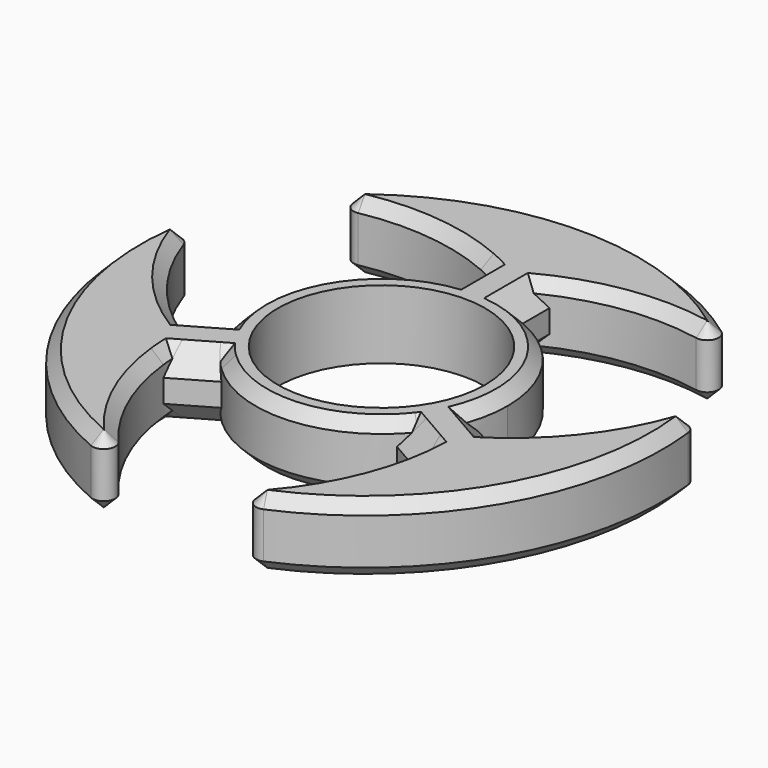
from build123d import *

# Parameters (mm, degrees)
F0_R          = 11.5
F1_DEPTH      = 7.62
F2_R          = 1.27
F3_SIZE       = 2.54
F4_T2_ANGLE   = 73.3947953897
F4_T4_ANGLE   = 73.3947953897
F4_T6_ANGLE   = 73.3947953897
F4_T8_ANGLE   = 73.3947953897
F4_T10_ANGLE  = 73.3947953897
F4_T12_ANGLE  = 73.3947953897
F4_T14_ANGLE  = 88.3467597363
F4_T16_ANGLE  = 88.3467597363
F4_T18_ANGLE  = 88.3467597363
F4_T20_ANGLE  = 88.3467597363
F4_T22_ANGLE  = 88.3467597363
F4_T24_ANGLE  = 88.3467597363
F4_T28_ANGLE  = 24.0059301026
F4_T33_ANGLE  = 24.0059301026
F4_T38_ANGLE  = 24.0059301026
F4_T43_ANGLE  = 24.0059301026
F4_T48_ANGLE  = 24.0059301026
F4_T53_ANGLE  = 24.0059301026
F4_T58_ANGLE  = 24.0059301026
F4_T63_ANGLE  = 24.0059301026
F4_T68_ANGLE  = 24.0059301026
F4_T73_ANGLE  = 24.0059301026
F4_T78_ANGLE  = 24.0059301026
F4_T83_ANGLE  = 24.0059301026
F4_T88_ANGLE  = 24.0059301026
F4_T93_ANGLE  = 24.0059301026
F4_T98_ANGLE  = 24.0059301026
F4_T103_ANGLE = 24.0059301026
F4_T108_ANGLE = 24.0059301026
F4_T113_ANGLE = 24.0059301026
F4_T118_ANGLE = 24.0059301026
F4_T123_ANGLE = 24.0059301026
F4_T128_ANGLE = 24.0059301026
F4_T133_ANGLE = 24.0059301026
F4_T138_ANGLE = 24.0059301026
F4_T143_ANGLE = 24.0059301026
F4_T146_ANGLE = 154.1156868675
F4_T148_ANGLE = 154.1156868949
F4_T150_ANGLE = 34.3912629475
F4_T154_ANGLE = 13.7891656583
F4_T157_ANGLE = 34.3912629475
F4_T161_ANGLE = 13.7891656583
F4_T164_ANGLE = 154.1156868675
F4_T166_ANGLE = 154.1156868675
F4_T168_ANGLE = 34.3912629475
F4_T172_ANGLE = 13.7891656583
F4_T175_ANGLE = 34.3912629475
F4_T179_ANGLE = 13.7891656583
F4_T182_ANGLE = 154.1156868675
F4_T184_ANGLE = 154.1156868675
F4_T186_ANGLE = 34.3912629475
F4_T190_ANGLE = 13.7891656583
F4_T193_ANGLE = 34.3912629475
F4_T197_ANGLE = 13.7891656583
F4_T200_ANGLE = 154.1156868675
F4_T202_ANGLE = 154.1156868949
F4_T204_ANGLE = 34.3912629475
F4_T208_ANGLE = 13.7891656583
F4_T211_ANGLE = 34.3912629475
F4_T215_ANGLE = 13.7891656583
F4_T218_ANGLE = 154.1156868675
F4_T220_ANGLE = 154.1156868675
F4_T222_ANGLE = 34.3912629475
F4_T226_ANGLE = 13.7891656583
F4_T229_ANGLE = 34.3912629475
F4_T233_ANGLE = 13.7891656583
F4_T236_ANGLE = 154.1156868675
F4_T238_ANGLE = 154.1156868675
F4_T240_ANGLE = 34.3912629475
F4_T244_ANGLE = 13.7891656583
F4_T247_ANGLE = 34.3912629475
F4_T251_ANGLE = 13.7891656583


# Not quite as in the source:
# - a fillet or chamfer that OpenCascade refuses, or shapes differently, is made with other operations: its cross-section is extruded or revolved along the edge and cut away or added


with BuildPart() as f1:
    # F0 (on Top) → F1 (new body)
    with BuildSketch(Plane.XY):
        with BuildLine():
            ThreePointArc((13.5447422652, -3.4206515417), (13.8632779213, -1.7234921751), (13.97, 0))
            ThreePointArc((13.97, 0), (11.144204772, 8.4242269675), (3.81, 13.4404166602))
            ThreePointArc((3.81, 13.4404166602), (0, 13.97), (-3.81, 13.4404166602))
            ThreePointArc((-3.81, 13.4404166602), (-12.0983748909, 6.985), (-13.5447422652, -3.4206515417))
            ThreePointArc((-13.5447422652, -3.4206515417), (-12.0983748909, -6.985), (-9.7347422652, -10.0197651185))
            ThreePointArc((-9.7347422652, -10.0197651185), (0, -13.97), (9.7347422652, -10.0197651185))
            ThreePointArc((9.7347422652, -10.0197651185), (12.0983748909, -6.985), (13.5447422652, -3.4206515417))
        make_face()
        Circle(F0_R, mode=Mode.SUBTRACT)
        with BuildLine():
            ThreePointArc((-9.7347422652, -10.0197651185), (-12.0983748909, -6.985), (-13.5447422652, -3.4206515417))
            Line((-13.5447422652, -3.4206515417), (-17.9441513164, -5.9606515417))
            ThreePointArc((-17.9441513164, -5.9606515417), (-24.8605715822, 1.777908826), (-28.1041513164, 11.6369846632))
            ThreePointArc((-28.1041513164, 11.6369846632), (-25.1148689402, -14.5000763433), (-3.9741513164, -30.1574013234))
            ThreePointArc((-3.9741513164, -30.1574013234), (-10.8905715822, -22.4188409558), (-14.1341513164, -12.5597651185))
            Line((-14.1341513164, -12.5597651185), (-9.7347422652, -10.0197651185))
        make_face()
        with BuildLine():
            ThreePointArc((-3.81, 13.4404166602), (0, 13.97), (3.81, 13.4404166602))
            Line((3.81, 13.4404166602), (3.81, 18.5204166602))
            ThreePointArc((3.81, 18.5204166602), (13.97, 20.6409321298), (24.13, 18.5204166602))
            ThreePointArc((24.13, 18.5204166602), (0, 29.0001526866), (-24.13, 18.5204166602))
            ThreePointArc((-24.13, 18.5204166602), (-13.97, 20.6409321298), (-3.81, 18.5204166602))
            Line((-3.81, 18.5204166602), (-3.81, 13.4404166602))
        make_face()
        with BuildLine():
            Line((17.9441513164, -5.9606515417), (13.5447422652, -3.4206515417))
            ThreePointArc((13.5447422652, -3.4206515417), (12.0983748909, -6.985), (9.7347422652, -10.0197651185))
            Line((9.7347422652, -10.0197651185), (14.1341513164, -12.5597651185))
            ThreePointArc((14.1341513164, -12.5597651185), (10.8905715822, -22.4188409558), (3.9741513164, -30.1574013234))
            ThreePointArc((3.9741513164, -30.1574013234), (25.1148689402, -14.5000763433), (28.1041513164, 11.6369846632))
            ThreePointArc((28.1041513164, 11.6369846632), (24.8605715822, 1.777908826), (17.9441513164, -5.9606515417))
        make_face()
    extrude(amount=F1_DEPTH)

    # F2
    f2_edges = [f1.edges().sort_by_distance(p)[0] for p in [
        (-3.974151, -30.157401, 3.81),
        (3.974151, -30.157401, 3.81),
        (28.104151, 11.636985, 3.81),
        (24.13, 18.520417, 3.81),
        (-24.13, 18.520417, 3.81),
        (-28.104151, 11.636985, 3.81),
    ]]
    fillet(f2_edges, radius=F2_R)

    # F3
    f3_edges = [f1.edges().sort_by_distance(p)[0] for p in [
        (-11.934447, -11.289765, 7.62),
        (-15.744447, -4.690652, 7.62),
        (-3.81, 15.980417, 7.62),
        (3.81, 15.980417, 7.62),
        (15.744447, -4.690652, 7.62),
        (11.934447, -11.289765, 7.62),
        (-11.934447, -11.289765, 0),
        (-15.744447, -4.690652, 0),
        (-3.81, 15.980417, 0),
        (3.81, 15.980417, 0),
        (15.744447, -4.690652, 0),
        (11.934447, -11.289765, 0),
    ]]
    chamfer(f3_edges, length=F3_SIZE)

    # F4: chamfer of 1.27 on 12 edges, made by hand

    # F4_s1 → F4_t2 (revolve, cut)
    with BuildSketch(Plane(origin=(-2.2062629319, -0.9502857256, 0), x_dir=(0, 0, 1), z_dir=(-0.9184284152, -0.3955872169, 0))):
        Polygon((0, -28.5268752215), (1.27, -29.7968752215), (0, -29.7968752215), align=None)
    revolve(axis=Axis((-3.4812898927, 2.0099236567, 0), (0, 0, 1)), revolution_arc=F4_T2_ANGLE, mode=Mode.SUBTRACT)

    # F4_s3 → F4_t4 (revolve, cut)
    with BuildSketch(Plane(origin=(1.9261030452, -1.4355368837, 0), x_dir=(0, 0, 1), z_dir=(0.8018027868, -0.5975887307, 0))):
        Polygon((0, -28.5268752215), (1.27, -29.7968752215), (0, -29.7968752215), align=None)
    revolve(axis=Axis((0, -4.0198473134, 0), (0, 0, 1)), revolution_arc=F4_T4_ANGLE, mode=Mode.SUBTRACT)

    # F4_s5 → F4_t6 (revolve, cut)
    with BuildSketch(Plane(origin=(0.2801598867, 2.3858226093, 0), x_dir=(0, 0, 1), z_dir=(0.1166256284, 0.9931759476, 0))):
        Polygon((0, -28.5268752215), (1.27, -29.7968752215), (0, -29.7968752215), align=None)
    revolve(axis=Axis((3.4812898927, 2.0099236567, 0), (0, 0, 1)), revolution_arc=F4_T6_ANGLE, mode=Mode.SUBTRACT)

    # F4_s7 → F4_t8 (revolve, cut)
    with BuildSketch(Plane(origin=(-2.2062629319, -0.9502857256, 0), x_dir=(0, 0, 1), z_dir=(-0.9184284152, -0.3955872169, 0))):
        Polygon((7.62, -28.5268752215), (6.35, -29.7968752215), (7.62, -29.7968752215), align=None)
    revolve(axis=Axis((-3.4812898927, 2.0099236567, 7.62), (0, 0, 1)), revolution_arc=F4_T8_ANGLE, mode=Mode.SUBTRACT)

    # F4_s9 → F4_t10 (revolve, cut)
    with BuildSketch(Plane(origin=(1.9261030452, -1.4355368837, 0), x_dir=(0, 0, 1), z_dir=(0.8018027868, -0.5975887307, 0))):
        Polygon((7.62, -28.5268752215), (6.35, -29.7968752215), (7.62, -29.7968752215), align=None)
    revolve(axis=Axis((0, -4.0198473134, 7.62), (0, 0, 1)), revolution_arc=F4_T10_ANGLE, mode=Mode.SUBTRACT)

    # F4_s11 → F4_t12 (revolve, cut)
    with BuildSketch(Plane(origin=(0.2801598867, 2.3858226093, 0), x_dir=(0, 0, 1), z_dir=(0.1166256284, 0.9931759476, 0))):
        Polygon((7.62, -28.5268752215), (6.35, -29.7968752215), (7.62, -29.7968752215), align=None)
    revolve(axis=Axis((3.4812898927, 2.0099236567, 7.62), (0, 0, 1)), revolution_arc=F4_T12_ANGLE, mode=Mode.SUBTRACT)

    # F4_s13 → F4_t14 (revolve, cut)
    with BuildSketch(Plane(origin=(0, 0, 0), x_dir=(0, 0, 1), z_dir=(-0.7172344394, 0.6968319445, 0))):
        Polygon((7.62, -12.7), (6.35, -13.97), (7.62, -13.97), align=None)
    revolve(axis=Axis((0, 0, 7.62), (0, 0, 1)), revolution_arc=F4_T14_ANGLE, mode=Mode.SUBTRACT)

    # F4_s15 → F4_t16 (revolve, cut)
    with BuildSketch(Plane(origin=(0, 0, 0), x_dir=(0, 0, 1), z_dir=(-0.2448569464, -0.9695592173, 0))):
        Polygon((7.62, -12.7), (6.35, -13.97), (7.62, -13.97), align=None)
    revolve(axis=Axis((0, 0, 7.62), (0, 0, 1)), revolution_arc=F4_T16_ANGLE, mode=Mode.SUBTRACT)

    # F4_s17 → F4_t18 (revolve, cut)
    with BuildSketch(Plane(origin=(0, 0, 0), x_dir=(0, 0, 1), z_dir=(0.9620913858, 0.2727272727, 0))):
        Polygon((7.62, -12.7), (6.35, -13.97), (7.62, -13.97), align=None)
    revolve(axis=Axis((0, 0, 7.62), (0, 0, 1)), revolution_arc=F4_T18_ANGLE, mode=Mode.SUBTRACT)

    # F4_s19 → F4_t20 (revolve, cut)
    with BuildSketch(Plane(origin=(0, 0, 0), x_dir=(0, 0, 1), z_dir=(0.9620913858, 0.2727272727, 0))):
        Polygon((0, -12.7), (1.27, -13.97), (0, -13.97), align=None)
    revolve(axis=Axis((0, 0, 0), (0, 0, 1)), revolution_arc=F4_T20_ANGLE, mode=Mode.SUBTRACT)

    # F4_s21 → F4_t22 (revolve, cut)
    with BuildSketch(Plane(origin=(0, 0, 0), x_dir=(0, 0, 1), z_dir=(-0.7172344394, 0.6968319445, 0))):
        Polygon((0, -12.7), (1.27, -13.97), (0, -13.97), align=None)
    revolve(axis=Axis((0, 0, 0), (0, 0, 1)), revolution_arc=F4_T22_ANGLE, mode=Mode.SUBTRACT)

    # F4_s23 → F4_t24 (revolve, cut)
    with BuildSketch(Plane(origin=(0, 0, 0), x_dir=(0, 0, 1), z_dir=(-0.2448569464, -0.9695592173, 0))):
        Polygon((0, -12.7), (1.27, -13.97), (0, -13.97), align=None)
    revolve(axis=Axis((0, 0, 0), (0, 0, 1)), revolution_arc=F4_T24_ANGLE, mode=Mode.SUBTRACT)


with BuildPart() as f4_tool26:
    # F4_s27 → F4_t28 (revolve)
    with BuildSketch(Plane(origin=(0, 0, 0), x_dir=(0, 0, 1), z_dir=(0.2448569464, 0.9695592173, 0))):
        Polygon((0, 12.7), (1.27, 13.97), (0, 13.97), align=None)
    revolve(axis=Axis((0, 0, 0), (0, 0, -1)), revolution_arc=F4_T28_ANGLE)

    split(bisect_by=Plane(origin=(0.3175, 0.5499261314, -0.635), x_dir=(-0.8660254038, 0.5, 0), z_dir=(0.3535533906, 0.6123724357, -0.7071067812)), keep=Keep.TOP)


with BuildPart() as f1_1:
    add(f1.part)

    # F4_t25: cut F4_tool26
    add(f4_tool26.part, mode=Mode.SUBTRACT)


with BuildPart() as f4_tool31:
    # F4_s32 → F4_t33 (revolve)
    with BuildSketch(Plane(origin=(0, 0, 0), x_dir=(0, 0, 1), z_dir=(0.2448569464, 0.9695592173, 0))):
        Polygon((0, 12.7), (1.27, 13.97), (0, 13.97), align=None)
    revolve(axis=Axis((0, 0, 0), (0, 0, -1)), revolution_arc=F4_T33_ANGLE)

    split(bisect_by=Plane(origin=(-0.3175, -0.5499261314, -0.635), x_dir=(0.8660254038, -0.5, 0), z_dir=(-0.3535533906, -0.6123724357, -0.7071067812)), keep=Keep.TOP)


with BuildPart() as f1_2:
    add(f1_1.part)

    # F4_t30: cut F4_tool31
    add(f4_tool31.part, mode=Mode.SUBTRACT)


with BuildPart() as f4_tool36:
    # F4_s37 → F4_t38 (revolve)
    with BuildSketch(Plane(origin=(0, 0, 0), x_dir=(0, 0, 1), z_dir=(0.9620913858, -0.2727272727, 0))):
        Polygon((0, -12.7), (1.27, -13.97), (0, -13.97), align=None)
    revolve(axis=Axis((0, 0, 0), (0, 0, 1)), revolution_arc=F4_T38_ANGLE)

    split(bisect_by=Plane(origin=(0.635, 0, -0.635), x_dir=(0, 1, 0), z_dir=(0.7071067812, 0, -0.7071067812)), keep=Keep.TOP)


with BuildPart() as f1_3:
    add(f1_2.part)

    # F4_t35: cut F4_tool36
    add(f4_tool36.part, mode=Mode.SUBTRACT)


with BuildPart() as f4_tool41:
    # F4_s42 → F4_t43 (revolve)
    with BuildSketch(Plane(origin=(0, 0, 0), x_dir=(0, 0, 1), z_dir=(0.9620913858, -0.2727272727, 0))):
        Polygon((0, -12.7), (1.27, -13.97), (0, -13.97), align=None)
    revolve(axis=Axis((0, 0, 0), (0, 0, 1)), revolution_arc=F4_T43_ANGLE)

    split(bisect_by=Plane(origin=(-0.635, 0, -0.635), x_dir=(0, 1, 0), z_dir=(-0.7071067812, 0, -0.7071067812)), keep=Keep.TOP)


with BuildPart() as f1_4:
    add(f1_3.part)

    # F4_t40: cut F4_tool41
    add(f4_tool41.part, mode=Mode.SUBTRACT)


with BuildPart() as f4_tool46:
    # F4_s47 → F4_t48 (revolve)
    with BuildSketch(Plane(origin=(0, 0, 0), x_dir=(0, 0, 1), z_dir=(0.7172344394, -0.6968319445, 0))):
        Polygon((0, 12.7), (1.27, 13.97), (0, 13.97), align=None)
    revolve(axis=Axis((0, 0, 0), (0, 0, -1)), revolution_arc=F4_T48_ANGLE)

    split(bisect_by=Plane(origin=(0.3175, -0.5499261314, -0.635), x_dir=(0.8660254038, 0.5, 0), z_dir=(0.3535533906, -0.6123724357, -0.7071067812)), keep=Keep.TOP)


with BuildPart() as f1_5:
    add(f1_4.part)

    # F4_t45: cut F4_tool46
    add(f4_tool46.part, mode=Mode.SUBTRACT)


with BuildPart() as f4_tool51:
    # F4_s52 → F4_t53 (revolve)
    with BuildSketch(Plane(origin=(0, 0, 0), x_dir=(0, 0, 1), z_dir=(0.7172344394, -0.6968319445, 0))):
        Polygon((0, 12.7), (1.27, 13.97), (0, 13.97), align=None)
    revolve(axis=Axis((0, 0, 0), (0, 0, -1)), revolution_arc=F4_T53_ANGLE)

    split(bisect_by=Plane(origin=(-0.3175, 0.5499261314, -0.635), x_dir=(-0.8660254038, -0.5, 0), z_dir=(-0.3535533906, 0.6123724357, -0.7071067812)), keep=Keep.TOP)


with BuildPart() as f1_6:
    add(f1_5.part)

    # F4_t50: cut F4_tool51
    add(f4_tool51.part, mode=Mode.SUBTRACT)


with BuildPart() as f4_tool56:
    # F4_s57 → F4_t58 (revolve)
    with BuildSketch(Plane(origin=(0, 0, 0), x_dir=(0, 0, 1), z_dir=(-0.7172344394, -0.6968319445, 0))):
        Polygon((0, -12.7), (1.27, -13.97), (0, -13.97), align=None)
    revolve(axis=Axis((0, 0, 0), (0, 0, 1)), revolution_arc=F4_T58_ANGLE)

    split(bisect_by=Plane(origin=(-0.3175, -0.5499261314, -0.635), x_dir=(0.8660254038, -0.5, 0), z_dir=(-0.3535533906, -0.6123724357, -0.7071067812)), keep=Keep.TOP)


with BuildPart() as f1_7:
    add(f1_6.part)

    # F4_t55: cut F4_tool56
    add(f4_tool56.part, mode=Mode.SUBTRACT)


with BuildPart() as f4_tool61:
    # F4_s62 → F4_t63 (revolve)
    with BuildSketch(Plane(origin=(0, 0, 0), x_dir=(0, 0, 1), z_dir=(-0.7172344394, -0.6968319445, 0))):
        Polygon((0, -12.7), (1.27, -13.97), (0, -13.97), align=None)
    revolve(axis=Axis((0, 0, 0), (0, 0, 1)), revolution_arc=F4_T63_ANGLE)

    split(bisect_by=Plane(origin=(0.3175, 0.5499261314, -0.635), x_dir=(-0.8660254038, 0.5, 0), z_dir=(0.3535533906, 0.6123724357, -0.7071067812)), keep=Keep.TOP)


with BuildPart() as f1_8:
    add(f1_7.part)

    # F4_t60: cut F4_tool61
    add(f4_tool61.part, mode=Mode.SUBTRACT)


with BuildPart() as f4_tool66:
    # F4_s67 → F4_t68 (revolve)
    with BuildSketch(Plane(origin=(0, 0, 0), x_dir=(0, 0, 1), z_dir=(-0.9620913858, -0.2727272727, 0))):
        Polygon((0, 12.7), (1.27, 13.97), (0, 13.97), align=None)
    revolve(axis=Axis((0, 0, 0), (0, 0, -1)), revolution_arc=F4_T68_ANGLE)

    split(bisect_by=Plane(origin=(-0.635, 0, -0.635), x_dir=(0, 1, 0), z_dir=(-0.7071067812, 0, -0.7071067812)), keep=Keep.TOP)


with BuildPart() as f1_9:
    add(f1_8.part)

    # F4_t65: cut F4_tool66
    add(f4_tool66.part, mode=Mode.SUBTRACT)


with BuildPart() as f4_tool71:
    # F4_s72 → F4_t73 (revolve)
    with BuildSketch(Plane(origin=(0, 0, 0), x_dir=(0, 0, 1), z_dir=(-0.9620913858, -0.2727272727, 0))):
        Polygon((0, 12.7), (1.27, 13.97), (0, 13.97), align=None)
    revolve(axis=Axis((0, 0, 0), (0, 0, -1)), revolution_arc=F4_T73_ANGLE)

    split(bisect_by=Plane(origin=(0.635, 0, -0.635), x_dir=(0, 1, 0), z_dir=(0.7071067812, 0, -0.7071067812)), keep=Keep.TOP)


with BuildPart() as f1_10:
    add(f1_9.part)

    # F4_t70: cut F4_tool71
    add(f4_tool71.part, mode=Mode.SUBTRACT)


with BuildPart() as f4_tool76:
    # F4_s77 → F4_t78 (revolve)
    with BuildSketch(Plane(origin=(0, 0, 0), x_dir=(0, 0, 1), z_dir=(-0.2448569464, 0.9695592173, 0))):
        Polygon((0, -12.7), (1.27, -13.97), (0, -13.97), align=None)
    revolve(axis=Axis((0, 0, 0), (0, 0, 1)), revolution_arc=F4_T78_ANGLE)

    split(bisect_by=Plane(origin=(-0.3175, 0.5499261314, -0.635), x_dir=(-0.8660254038, -0.5, 0), z_dir=(-0.3535533906, 0.6123724357, -0.7071067812)), keep=Keep.TOP)


with BuildPart() as f1_11:
    add(f1_10.part)

    # F4_t75: cut F4_tool76
    add(f4_tool76.part, mode=Mode.SUBTRACT)


with BuildPart() as f4_tool81:
    # F4_s82 → F4_t83 (revolve)
    with BuildSketch(Plane(origin=(0, 0, 0), x_dir=(0, 0, 1), z_dir=(-0.2448569464, 0.9695592173, 0))):
        Polygon((0, -12.7), (1.27, -13.97), (0, -13.97), align=None)
    revolve(axis=Axis((0, 0, 0), (0, 0, 1)), revolution_arc=F4_T83_ANGLE)

    split(bisect_by=Plane(origin=(0.3175, -0.5499261314, -0.635), x_dir=(0.8660254038, 0.5, 0), z_dir=(0.3535533906, -0.6123724357, -0.7071067812)), keep=Keep.TOP)


with BuildPart() as f1_12:
    add(f1_11.part)

    # F4_t80: cut F4_tool81
    add(f4_tool81.part, mode=Mode.SUBTRACT)


with BuildPart() as f4_tool86:
    # F4_s87 → F4_t88 (revolve)
    with BuildSketch(Plane(origin=(0, 0, 0), x_dir=(0, 0, 1), z_dir=(-0.9620913858, -0.2727272727, 0))):
        Polygon((7.62, 12.7), (6.35, 13.97), (7.62, 13.97), align=None)
    revolve(axis=Axis((0, 0, 7.62), (0, 0, -1)), revolution_arc=F4_T88_ANGLE)

    split(bisect_by=Plane(origin=(-4.445, 0, 4.445), x_dir=(0, 1, 0), z_dir=(-0.7071067812, 0, 0.7071067812)), keep=Keep.TOP)


with BuildPart() as f1_13:
    add(f1_12.part)

    # F4_t85: cut F4_tool86
    add(f4_tool86.part, mode=Mode.SUBTRACT)


with BuildPart() as f4_tool91:
    # F4_s92 → F4_t93 (revolve)
    with BuildSketch(Plane(origin=(0, 0, 0), x_dir=(0, 0, 1), z_dir=(-0.9620913858, -0.2727272727, 0))):
        Polygon((7.62, 12.7), (6.35, 13.97), (7.62, 13.97), align=None)
    revolve(axis=Axis((0, 0, 7.62), (0, 0, -1)), revolution_arc=F4_T93_ANGLE)

    split(bisect_by=Plane(origin=(4.445, 0, 4.445), x_dir=(0, 1, 0), z_dir=(0.7071067812, 0, 0.7071067812)), keep=Keep.TOP)


with BuildPart() as f1_14:
    add(f1_13.part)

    # F4_t90: cut F4_tool91
    add(f4_tool91.part, mode=Mode.SUBTRACT)


with BuildPart() as f4_tool96:
    # F4_s97 → F4_t98 (revolve)
    with BuildSketch(Plane(origin=(0, 0, 0), x_dir=(0, 0, 1), z_dir=(-0.2448569464, 0.9695592173, 0))):
        Polygon((7.62, -12.7), (6.35, -13.97), (7.62, -13.97), align=None)
    revolve(axis=Axis((0, 0, 7.62), (0, 0, 1)), revolution_arc=F4_T98_ANGLE)

    split(bisect_by=Plane(origin=(-2.2225, 3.8494829198, 4.445), x_dir=(-0.8660254038, -0.5, 0), z_dir=(-0.3535533906, 0.6123724357, 0.7071067812)), keep=Keep.TOP)


with BuildPart() as f1_15:
    add(f1_14.part)

    # F4_t95: cut F4_tool96
    add(f4_tool96.part, mode=Mode.SUBTRACT)


with BuildPart() as f4_tool101:
    # F4_s102 → F4_t103 (revolve)
    with BuildSketch(Plane(origin=(0, 0, 0), x_dir=(0, 0, 1), z_dir=(-0.2448569464, 0.9695592173, 0))):
        Polygon((7.62, -12.7), (6.35, -13.97), (7.62, -13.97), align=None)
    revolve(axis=Axis((0, 0, 7.62), (0, 0, 1)), revolution_arc=F4_T103_ANGLE)

    split(bisect_by=Plane(origin=(2.2225, -3.8494829198, 4.445), x_dir=(0.8660254038, 0.5, 0), z_dir=(0.3535533906, -0.6123724357, 0.7071067812)), keep=Keep.TOP)


with BuildPart() as f1_16:
    add(f1_15.part)

    # F4_t100: cut F4_tool101
    add(f4_tool101.part, mode=Mode.SUBTRACT)


with BuildPart() as f4_tool106:
    # F4_s107 → F4_t108 (revolve)
    with BuildSketch(Plane(origin=(0, 0, 0), x_dir=(0, 0, 1), z_dir=(0.2448569464, 0.9695592173, 0))):
        Polygon((7.62, 12.7), (6.35, 13.97), (7.62, 13.97), align=None)
    revolve(axis=Axis((0, 0, 7.62), (0, 0, -1)), revolution_arc=F4_T108_ANGLE)

    split(bisect_by=Plane(origin=(2.2225, 3.8494829198, 4.445), x_dir=(-0.8660254038, 0.5, 0), z_dir=(0.3535533906, 0.6123724357, 0.7071067812)), keep=Keep.TOP)


with BuildPart() as f1_17:
    add(f1_16.part)

    # F4_t105: cut F4_tool106
    add(f4_tool106.part, mode=Mode.SUBTRACT)


with BuildPart() as f4_tool111:
    # F4_s112 → F4_t113 (revolve)
    with BuildSketch(Plane(origin=(0, 0, 0), x_dir=(0, 0, 1), z_dir=(0.2448569464, 0.9695592173, 0))):
        Polygon((7.62, 12.7), (6.35, 13.97), (7.62, 13.97), align=None)
    revolve(axis=Axis((0, 0, 7.62), (0, 0, -1)), revolution_arc=F4_T113_ANGLE)

    split(bisect_by=Plane(origin=(-2.2225, -3.8494829198, 4.445), x_dir=(0.8660254038, -0.5, 0), z_dir=(-0.3535533906, -0.6123724357, 0.7071067812)), keep=Keep.TOP)


with BuildPart() as f1_18:
    add(f1_17.part)

    # F4_t110: cut F4_tool111
    add(f4_tool111.part, mode=Mode.SUBTRACT)


with BuildPart() as f4_tool116:
    # F4_s117 → F4_t118 (revolve)
    with BuildSketch(Plane(origin=(0, 0, 0), x_dir=(0, 0, 1), z_dir=(0.9620913858, -0.2727272727, 0))):
        Polygon((7.62, -12.7), (6.35, -13.97), (7.62, -13.97), align=None)
    revolve(axis=Axis((0, 0, 7.62), (0, 0, 1)), revolution_arc=F4_T118_ANGLE)

    split(bisect_by=Plane(origin=(4.445, 0, 4.445), x_dir=(0, 1, 0), z_dir=(0.7071067812, 0, 0.7071067812)), keep=Keep.TOP)


with BuildPart() as f1_19:
    add(f1_18.part)

    # F4_t115: cut F4_tool116
    add(f4_tool116.part, mode=Mode.SUBTRACT)


with BuildPart() as f4_tool121:
    # F4_s122 → F4_t123 (revolve)
    with BuildSketch(Plane(origin=(0, 0, 0), x_dir=(0, 0, 1), z_dir=(0.9620913858, -0.2727272727, 0))):
        Polygon((7.62, -12.7), (6.35, -13.97), (7.62, -13.97), align=None)
    revolve(axis=Axis((0, 0, 7.62), (0, 0, 1)), revolution_arc=F4_T123_ANGLE)

    split(bisect_by=Plane(origin=(-4.445, 0, 4.445), x_dir=(0, 1, 0), z_dir=(-0.7071067812, 0, 0.7071067812)), keep=Keep.TOP)


with BuildPart() as f1_20:
    add(f1_19.part)

    # F4_t120: cut F4_tool121
    add(f4_tool121.part, mode=Mode.SUBTRACT)


with BuildPart() as f4_tool126:
    # F4_s127 → F4_t128 (revolve)
    with BuildSketch(Plane(origin=(0, 0, 0), x_dir=(0, 0, 1), z_dir=(0.7172344394, -0.6968319445, 0))):
        Polygon((7.62, 12.7), (6.35, 13.97), (7.62, 13.97), align=None)
    revolve(axis=Axis((0, 0, 7.62), (0, 0, -1)), revolution_arc=F4_T128_ANGLE)

    split(bisect_by=Plane(origin=(2.2225, -3.8494829198, 4.445), x_dir=(0.8660254038, 0.5, 0), z_dir=(0.3535533906, -0.6123724357, 0.7071067812)), keep=Keep.TOP)


with BuildPart() as f1_21:
    add(f1_20.part)

    # F4_t125: cut F4_tool126
    add(f4_tool126.part, mode=Mode.SUBTRACT)


with BuildPart() as f4_tool131:
    # F4_s132 → F4_t133 (revolve)
    with BuildSketch(Plane(origin=(0, 0, 0), x_dir=(0, 0, 1), z_dir=(0.7172344394, -0.6968319445, 0))):
        Polygon((7.62, 12.7), (6.35, 13.97), (7.62, 13.97), align=None)
    revolve(axis=Axis((0, 0, 7.62), (0, 0, -1)), revolution_arc=F4_T133_ANGLE)

    split(bisect_by=Plane(origin=(-2.2225, 3.8494829198, 4.445), x_dir=(-0.8660254038, -0.5, 0), z_dir=(-0.3535533906, 0.6123724357, 0.7071067812)), keep=Keep.TOP)


with BuildPart() as f1_22:
    add(f1_21.part)

    # F4_t130: cut F4_tool131
    add(f4_tool131.part, mode=Mode.SUBTRACT)


with BuildPart() as f4_tool136:
    # F4_s137 → F4_t138 (revolve)
    with BuildSketch(Plane(origin=(0, 0, 0), x_dir=(0, 0, 1), z_dir=(-0.7172344394, -0.6968319445, 0))):
        Polygon((7.62, -12.7), (6.35, -13.97), (7.62, -13.97), align=None)
    revolve(axis=Axis((0, 0, 7.62), (0, 0, 1)), revolution_arc=F4_T138_ANGLE)

    split(bisect_by=Plane(origin=(-2.2225, -3.8494829198, 4.445), x_dir=(0.8660254038, -0.5, 0), z_dir=(-0.3535533906, -0.6123724357, 0.7071067812)), keep=Keep.TOP)


with BuildPart() as f1_23:
    add(f1_22.part)

    # F4_t135: cut F4_tool136
    add(f4_tool136.part, mode=Mode.SUBTRACT)


with BuildPart() as f4_tool141:
    # F4_s142 → F4_t143 (revolve)
    with BuildSketch(Plane(origin=(0, 0, 0), x_dir=(0, 0, 1), z_dir=(-0.7172344394, -0.6968319445, 0))):
        Polygon((7.62, -12.7), (6.35, -13.97), (7.62, -13.97), align=None)
    revolve(axis=Axis((0, 0, 7.62), (0, 0, 1)), revolution_arc=F4_T143_ANGLE)

    split(bisect_by=Plane(origin=(2.2225, 3.8494829198, 4.445), x_dir=(-0.8660254038, 0.5, 0), z_dir=(0.3535533906, 0.6123724357, 0.7071067812)), keep=Keep.TOP)


with BuildPart() as f1_24:
    add(f1_23.part)

    # F4_t140: cut F4_tool141
    add(f4_tool141.part, mode=Mode.SUBTRACT)

    # F4_s145 → F4_t146 (revolve, cut)
    with BuildSketch(Plane(origin=(-4.8031625371, 13.8029526387, 0), x_dir=(0, 0, 1), z_dir=(0.3286509729, -0.9444514482, 0))):
        Polygon((7.62, 24.6162827639), (6.35, 23.3462827648), (7.62, 23.3462827639), align=None)
    revolve(axis=Axis((-28.0520464423, 5.7127873584, 7.62), (0, 0, 1)), revolution_arc=F4_T146_ANGLE, mode=Mode.SUBTRACT)

    # F4_s147 → F4_t148 (revolve, cut)
    with BuildSketch(Plane(origin=(2.2062629587, -0.9502857398, 0), x_dir=(0, 0, 1), z_dir=(-0.9184284148, 0.3955872178, 0))):
        Polygon((7.62, -28.5268752191), (6.35, -29.7968752182), (7.62, -29.7968752191), align=None)
    revolve(axis=Axis((-9.0786042423, -27.1501785268, 7.62), (0, 0, 1)), revolution_arc=F4_T148_ANGLE, mode=Mode.SUBTRACT)

    # F4_s149 → F4_t150 (revolve, cut)
    with BuildSketch(Plane(origin=(9.5521263672, -11.0611371171, 0), x_dir=(0, 0, 1), z_dir=(0.6535934597, -0.7568458162, 0))):
        Polygon((7.62, 24.6162827521), (6.35, 23.3462827521), (7.62, 23.3462827521), align=None)
    revolve(axis=Axis((11.1064736739, -9.7188409558, 7.62), (0, 0, -1)), revolution_arc=F4_T150_ANGLE, mode=Mode.SUBTRACT)


with BuildPart() as f4_tool152:
    # F4_s153 → F4_t154 (revolve)
    with BuildSketch(Plane(origin=(1.2191467399, -10.8316955702, 0), x_dir=(0, 0, 1), z_dir=(0.111847408, -0.9937253933, 0))):
        Polygon((7.62, 16.7202422495), (6.35, 15.4502422495), (7.62, 15.4502422495), align=None)
    revolve(axis=Axis((11.1064736739, -9.7188409558, 7.62), (0, 0, -1)), revolution_arc=F4_T154_ANGLE)

    split(bisect_by=Plane(origin=(2.2225, -3.8494829198, 4.445), x_dir=(0.8660254038, 0.5, 0), z_dir=(0.3535533906, -0.6123724357, 0.7071067812)), keep=Keep.TOP)


with BuildPart() as f1_25:
    add(f1_24.part)

    # F4_t151: cut F4_tool152
    add(f4_tool152.part, mode=Mode.SUBTRACT)

    # F4_s156 → F4_t157 (revolve, cut)
    with BuildSketch(Plane(origin=(-8.7709501599, 6.4716598328, 0), x_dir=(0, 0, 1), z_dir=(0.804667731, -0.5937253933, 0))):
        Polygon((7.62, 16.7202422495), (6.35, 15.4502422495), (7.62, 15.4502422495), align=None)
    revolve(axis=Axis((-2.8635263261, 14.477908826, 7.62), (0, 0, -1)), revolution_arc=F4_T157_ANGLE, mode=Mode.SUBTRACT)


with BuildPart() as f4_tool159:
    # F4_s160 → F4_t161 (revolve)
    with BuildSketch(Plane(origin=(-8.7709501599, 6.4716598328, 0), x_dir=(0, 0, 1), z_dir=(-0.804667731, 0.5937253933, 0))):
        Polygon((7.62, -16.7202422495), (6.35, -15.4502422495), (7.62, -15.4502422495), align=None)
    revolve(axis=Axis((-2.8635263261, 14.477908826, 7.62), (0, 0, 1)), revolution_arc=F4_T161_ANGLE)

    split(bisect_by=Plane(origin=(-2.2225, 3.8494829198, 4.445), x_dir=(-0.8660254038, -0.5, 0), z_dir=(-0.3535533906, 0.6123724357, 0.7071067812)), keep=Keep.TOP)


with BuildPart() as f1_26:
    add(f1_25.part)

    # F4_t158: cut F4_tool159
    add(f4_tool159.part, mode=Mode.SUBTRACT)

    # F4_s163 → F4_t164 (revolve, cut)
    with BuildSketch(Plane(origin=(14.3552889009, -2.7418155437, 0), x_dir=(0, 0, 1), z_dir=(-0.9822444332, 0.1876056326, 0))):
        Polygon((7.62, 24.6162827639), (6.35, 23.3462827648), (7.62, 23.3462827639), align=None)
    revolve(axis=Axis((18.9734422, 21.437391168, 7.62), (0, 0, 1)), revolution_arc=F4_T164_ANGLE, mode=Mode.SUBTRACT)

    # F4_s165 → F4_t166 (revolve, cut)
    with BuildSketch(Plane(origin=(-1.9261030658, -1.4355368966, 0), x_dir=(0, 0, 1), z_dir=(0.8018027873, 0.59758873, 0))):
        Polygon((7.62, -28.5268752195), (6.35, -29.7968752187), (7.62, -29.7968752195), align=None)
    revolve(axis=Axis((-18.9734422, 21.437391168, 7.62), (0, 0, 1)), revolution_arc=F4_T166_ANGLE, mode=Mode.SUBTRACT)

    # F4_s167 → F4_t168 (revolve, cut)
    with BuildSketch(Plane(origin=(-14.3552889218, -2.7418155356, 0), x_dir=(0, 0, 1), z_dir=(-0.9822444334, -0.1876056318, 0))):
        Polygon((7.62, 24.6162827521), (6.35, 23.3462827521), (7.62, 23.3462827521), align=None)
    revolve(axis=Axis((-13.97, -4.7590678702, 7.62), (0, 0, -1)), revolution_arc=F4_T168_ANGLE, mode=Mode.SUBTRACT)


with BuildPart() as f4_tool170:
    # F4_s171 → F4_t172 (revolve)
    with BuildSketch(Plane(origin=(-9.9900968998, 4.3600357375, 0), x_dir=(0, 0, 1), z_dir=(-0.916515139, 0.4, 0))):
        Polygon((7.62, 16.7202422495), (6.35, 15.4502422495), (7.62, 15.4502422495), align=None)
    revolve(axis=Axis((-13.97, -4.7590678702, 7.62), (0, 0, -1)), revolution_arc=F4_T172_ANGLE)

    split(bisect_by=Plane(origin=(-4.445, 0, 4.445), x_dir=(0, 1, 0), z_dir=(-0.7071067812, 0, 0.7071067812)), keep=Keep.TOP)


with BuildPart() as f1_27:
    add(f1_26.part)

    # F4_t169: cut F4_tool170
    add(f4_tool170.part, mode=Mode.SUBTRACT)

    # F4_s174 → F4_t175 (revolve, cut)
    with BuildSketch(Plane(origin=(9.9900968998, 4.3600357375, 0), x_dir=(0, 0, 1), z_dir=(-0.916515139, -0.4, 0))):
        Polygon((7.62, 16.7202422495), (6.35, 15.4502422495), (7.62, 15.4502422495), align=None)
    revolve(axis=Axis((13.97, -4.7590678702, 7.62), (0, 0, -1)), revolution_arc=F4_T175_ANGLE, mode=Mode.SUBTRACT)


with BuildPart() as f4_tool177:
    # F4_s178 → F4_t179 (revolve)
    with BuildSketch(Plane(origin=(9.9900968998, 4.3600357375, 0), x_dir=(0, 0, 1), z_dir=(0.916515139, 0.4, 0))):
        Polygon((7.62, -16.7202422495), (6.35, -15.4502422495), (7.62, -15.4502422495), align=None)
    revolve(axis=Axis((13.97, -4.7590678702, 7.62), (0, 0, 1)), revolution_arc=F4_T179_ANGLE)

    split(bisect_by=Plane(origin=(4.445, 0, 4.445), x_dir=(0, 1, 0), z_dir=(0.7071067812, 0, 0.7071067812)), keep=Keep.TOP)


with BuildPart() as f1_28:
    add(f1_27.part)

    # F4_t176: cut F4_tool177
    add(f4_tool177.part, mode=Mode.SUBTRACT)

    # F4_s181 → F4_t182 (revolve, cut)
    with BuildSketch(Plane(origin=(-9.5521263638, -11.061137095, 0), x_dir=(0, 0, 1), z_dir=(0.6535934603, 0.7568458156, 0))):
        Polygon((7.62, 24.6162827639), (6.35, 23.3462827648), (7.62, 23.3462827639), align=None)
    revolve(axis=Axis((9.0786042424, -27.1501785264, 7.62), (0, 0, 1)), revolution_arc=F4_T182_ANGLE, mode=Mode.SUBTRACT)

    # F4_s183 → F4_t184 (revolve, cut)
    with BuildSketch(Plane(origin=(-0.2801598876, 2.3858226336, 0), x_dir=(0, 0, 1), z_dir=(0.1166256276, -0.9931759477, 0))):
        Polygon((7.62, -28.5268752195), (6.35, -29.7968752187), (7.62, -29.7968752195), align=None)
    revolve(axis=Axis((28.0520464423, 5.7127873584, 7.62), (0, 0, 1)), revolution_arc=F4_T184_ANGLE, mode=Mode.SUBTRACT)

    # F4_s185 → F4_t186 (revolve, cut)
    with BuildSketch(Plane(origin=(4.8031625545, 13.8029526527, 0), x_dir=(0, 0, 1), z_dir=(0.3286509737, 0.9444514479, 0))):
        Polygon((7.62, 24.6162827521), (6.35, 23.3462827521), (7.62, 23.3462827521), align=None)
    revolve(axis=Axis((2.8635263261, 14.477908826, 7.62), (0, 0, -1)), revolution_arc=F4_T186_ANGLE, mode=Mode.SUBTRACT)


with BuildPart() as f4_tool188:
    # F4_s189 → F4_t190 (revolve)
    with BuildSketch(Plane(origin=(8.7709501599, 6.4716598328, 0), x_dir=(0, 0, 1), z_dir=(0.804667731, 0.5937253933, 0))):
        Polygon((7.62, 16.7202422495), (6.35, 15.4502422495), (7.62, 15.4502422495), align=None)
    revolve(axis=Axis((2.8635263261, 14.477908826, 7.62), (0, 0, -1)), revolution_arc=F4_T190_ANGLE)

    split(bisect_by=Plane(origin=(2.2225, 3.8494829198, 4.445), x_dir=(-0.8660254038, 0.5, 0), z_dir=(0.3535533906, 0.6123724357, 0.7071067812)), keep=Keep.TOP)


with BuildPart() as f1_29:
    add(f1_28.part)

    # F4_t187: cut F4_tool188
    add(f4_tool188.part, mode=Mode.SUBTRACT)

    # F4_s192 → F4_t193 (revolve, cut)
    with BuildSketch(Plane(origin=(-1.2191467399, -10.8316955702, 0), x_dir=(0, 0, 1), z_dir=(0.111847408, 0.9937253933, 0))):
        Polygon((6.35, 15.4502422495), (7.62, 16.7202422495), (7.62, 15.4502422495), align=None)
    revolve(axis=Axis((-11.1064736739, -9.7188409558, 7.62), (0, 0, -1)), revolution_arc=F4_T193_ANGLE, mode=Mode.SUBTRACT)


with BuildPart() as f4_tool195:
    # F4_s196 → F4_t197 (revolve)
    with BuildSketch(Plane(origin=(-1.2191467399, -10.8316955702, 0), x_dir=(0, 0, 1), z_dir=(-0.111847408, -0.9937253933, 0))):
        Polygon((6.35, -15.4502422495), (7.62, -16.7202422495), (7.62, -15.4502422495), align=None)
    revolve(axis=Axis((-11.1064736739, -9.7188409558, 7.62), (0, 0, 1)), revolution_arc=F4_T197_ANGLE)

    split(bisect_by=Plane(origin=(-2.2225, -3.8494829198, 4.445), x_dir=(0.8660254038, -0.5, 0), z_dir=(-0.3535533906, -0.6123724357, 0.7071067812)), keep=Keep.TOP)


with BuildPart() as f1_30:
    add(f1_29.part)

    # F4_t194: cut F4_tool195
    add(f4_tool195.part, mode=Mode.SUBTRACT)

    # F4_s199 → F4_t200 (revolve, cut)
    with BuildSketch(Plane(origin=(-4.8031625371, 13.8029526387, 0), x_dir=(0, 0, 1), z_dir=(0.3286509729, -0.9444514482, 0))):
        Polygon((0, 24.6162827639), (1.27, 23.3462827648), (0, 23.3462827639), align=None)
    revolve(axis=Axis((-28.0520464423, 5.7127873584, 0), (0, 0, 1)), revolution_arc=F4_T200_ANGLE, mode=Mode.SUBTRACT)

    # F4_s201 → F4_t202 (revolve, cut)
    with BuildSketch(Plane(origin=(2.2062629587, -0.9502857398, 0), x_dir=(0, 0, 1), z_dir=(-0.9184284148, 0.3955872178, 0))):
        Polygon((0, -28.5268752191), (1.27, -29.7968752182), (0, -29.7968752191), align=None)
    revolve(axis=Axis((-9.0786042423, -27.1501785268, 0), (0, 0, 1)), revolution_arc=F4_T202_ANGLE, mode=Mode.SUBTRACT)

    # F4_s203 → F4_t204 (revolve, cut)
    with BuildSketch(Plane(origin=(9.5521263672, -11.0611371171, 0), x_dir=(0, 0, 1), z_dir=(0.6535934597, -0.7568458162, 0))):
        Polygon((0, 24.6162827521), (1.27, 23.3462827521), (0, 23.3462827521), align=None)
    revolve(axis=Axis((11.1064736739, -9.7188409558, 0), (0, 0, -1)), revolution_arc=F4_T204_ANGLE, mode=Mode.SUBTRACT)


with BuildPart() as f4_tool206:
    # F4_s207 → F4_t208 (revolve)
    with BuildSketch(Plane(origin=(1.2191467399, -10.8316955702, 0), x_dir=(0, 0, 1), z_dir=(0.111847408, -0.9937253933, 0))):
        Polygon((0, 16.7202422495), (1.27, 15.4502422495), (0, 15.4502422495), align=None)
    revolve(axis=Axis((11.1064736739, -9.7188409558, 0), (0, 0, -1)), revolution_arc=F4_T208_ANGLE)

    split(bisect_by=Plane(origin=(0.3175, -0.5499261314, -0.635), x_dir=(0.8660254038, 0.5, 0), z_dir=(0.3535533906, -0.6123724357, -0.7071067812)), keep=Keep.TOP)


with BuildPart() as f1_31:
    add(f1_30.part)

    # F4_t205: cut F4_tool206
    add(f4_tool206.part, mode=Mode.SUBTRACT)

    # F4_s210 → F4_t211 (revolve, cut)
    with BuildSketch(Plane(origin=(-8.7709501599, 6.4716598328, 0), x_dir=(0, 0, 1), z_dir=(0.804667731, -0.5937253933, 0))):
        Polygon((0, 16.7202422495), (1.27, 15.4502422495), (0, 15.4502422495), align=None)
    revolve(axis=Axis((-2.8635263261, 14.477908826, 0), (0, 0, -1)), revolution_arc=F4_T211_ANGLE, mode=Mode.SUBTRACT)


with BuildPart() as f4_tool213:
    # F4_s214 → F4_t215 (revolve)
    with BuildSketch(Plane(origin=(-8.7709501599, 6.4716598328, 0), x_dir=(0, 0, 1), z_dir=(-0.804667731, 0.5937253933, 0))):
        Polygon((0, -16.7202422495), (1.27, -15.4502422495), (0, -15.4502422495), align=None)
    revolve(axis=Axis((-2.8635263261, 14.477908826, 0), (0, 0, 1)), revolution_arc=F4_T215_ANGLE)

    split(bisect_by=Plane(origin=(-0.3175, 0.5499261314, -0.635), x_dir=(-0.8660254038, -0.5, 0), z_dir=(-0.3535533906, 0.6123724357, -0.7071067812)), keep=Keep.TOP)


with BuildPart() as f1_32:
    add(f1_31.part)

    # F4_t212: cut F4_tool213
    add(f4_tool213.part, mode=Mode.SUBTRACT)

    # F4_s217 → F4_t218 (revolve, cut)
    with BuildSketch(Plane(origin=(14.3552889009, -2.7418155437, 0), x_dir=(0, 0, 1), z_dir=(-0.9822444332, 0.1876056326, 0))):
        Polygon((0, 24.6162827639), (1.27, 23.3462827648), (0, 23.3462827639), align=None)
    revolve(axis=Axis((18.9734422, 21.437391168, 0), (0, 0, 1)), revolution_arc=F4_T218_ANGLE, mode=Mode.SUBTRACT)

    # F4_s219 → F4_t220 (revolve, cut)
    with BuildSketch(Plane(origin=(-1.9261030658, -1.4355368966, 0), x_dir=(0, 0, 1), z_dir=(0.8018027873, 0.59758873, 0))):
        Polygon((0, -28.5268752195), (1.27, -29.7968752187), (0, -29.7968752195), align=None)
    revolve(axis=Axis((-18.9734422, 21.437391168, 0), (0, 0, 1)), revolution_arc=F4_T220_ANGLE, mode=Mode.SUBTRACT)

    # F4_s221 → F4_t222 (revolve, cut)
    with BuildSketch(Plane(origin=(-14.3552889218, -2.7418155356, 0), x_dir=(0, 0, 1), z_dir=(-0.9822444334, -0.1876056318, 0))):
        Polygon((0, 24.6162827521), (1.27, 23.3462827521), (0, 23.3462827521), align=None)
    revolve(axis=Axis((-13.97, -4.7590678702, 0), (0, 0, -1)), revolution_arc=F4_T222_ANGLE, mode=Mode.SUBTRACT)


with BuildPart() as f4_tool224:
    # F4_s225 → F4_t226 (revolve)
    with BuildSketch(Plane(origin=(-9.9900968998, 4.3600357375, 0), x_dir=(0, 0, 1), z_dir=(-0.916515139, 0.4, 0))):
        Polygon((0, 16.7202422495), (1.27, 15.4502422495), (0, 15.4502422495), align=None)
    revolve(axis=Axis((-13.97, -4.7590678702, 0), (0, 0, -1)), revolution_arc=F4_T226_ANGLE)

    split(bisect_by=Plane(origin=(-0.635, 0, -0.635), x_dir=(0, 1, 0), z_dir=(-0.7071067812, 0, -0.7071067812)), keep=Keep.TOP)


with BuildPart() as f1_33:
    add(f1_32.part)

    # F4_t223: cut F4_tool224
    add(f4_tool224.part, mode=Mode.SUBTRACT)

    # F4_s228 → F4_t229 (revolve, cut)
    with BuildSketch(Plane(origin=(9.9900968998, 4.3600357375, 0), x_dir=(0, 0, 1), z_dir=(-0.916515139, -0.4, 0))):
        Polygon((0, 16.7202422495), (1.27, 15.4502422495), (0, 15.4502422495), align=None)
    revolve(axis=Axis((13.97, -4.7590678702, 0), (0, 0, -1)), revolution_arc=F4_T229_ANGLE, mode=Mode.SUBTRACT)


with BuildPart() as f4_tool231:
    # F4_s232 → F4_t233 (revolve)
    with BuildSketch(Plane(origin=(9.9900968998, 4.3600357375, 0), x_dir=(0, 0, 1), z_dir=(0.916515139, 0.4, 0))):
        Polygon((0, -16.7202422495), (1.27, -15.4502422495), (0, -15.4502422495), align=None)
    revolve(axis=Axis((13.97, -4.7590678702, 0), (0, 0, 1)), revolution_arc=F4_T233_ANGLE)

    split(bisect_by=Plane(origin=(0.635, 0, -0.635), x_dir=(0, 1, 0), z_dir=(0.7071067812, 0, -0.7071067812)), keep=Keep.TOP)


with BuildPart() as f1_34:
    add(f1_33.part)

    # F4_t230: cut F4_tool231
    add(f4_tool231.part, mode=Mode.SUBTRACT)

    # F4_s235 → F4_t236 (revolve, cut)
    with BuildSketch(Plane(origin=(-9.5521263638, -11.061137095, 0), x_dir=(0, 0, 1), z_dir=(0.6535934603, 0.7568458156, 0))):
        Polygon((0, 24.6162827639), (1.27, 23.3462827648), (0, 23.3462827639), align=None)
    revolve(axis=Axis((9.0786042424, -27.1501785264, 0), (0, 0, 1)), revolution_arc=F4_T236_ANGLE, mode=Mode.SUBTRACT)

    # F4_s237 → F4_t238 (revolve, cut)
    with BuildSketch(Plane(origin=(-0.2801598876, 2.3858226336, 0), x_dir=(0, 0, 1), z_dir=(0.1166256276, -0.9931759477, 0))):
        Polygon((0, -28.5268752195), (1.27, -29.7968752187), (0, -29.7968752195), align=None)
    revolve(axis=Axis((28.0520464423, 5.7127873584, 0), (0, 0, 1)), revolution_arc=F4_T238_ANGLE, mode=Mode.SUBTRACT)

    # F4_s239 → F4_t240 (revolve, cut)
    with BuildSketch(Plane(origin=(4.8031625545, 13.8029526527, 0), x_dir=(0, 0, 1), z_dir=(0.3286509737, 0.9444514479, 0))):
        Polygon((0, 24.6162827521), (1.27, 23.3462827521), (0, 23.3462827521), align=None)
    revolve(axis=Axis((2.8635263261, 14.477908826, 0), (0, 0, -1)), revolution_arc=F4_T240_ANGLE, mode=Mode.SUBTRACT)


with BuildPart() as f4_tool242:
    # F4_s243 → F4_t244 (revolve)
    with BuildSketch(Plane(origin=(8.7709501599, 6.4716598328, 0), x_dir=(0, 0, 1), z_dir=(0.804667731, 0.5937253933, 0))):
        Polygon((0, 16.7202422495), (1.27, 15.4502422495), (0, 15.4502422495), align=None)
    revolve(axis=Axis((2.8635263261, 14.477908826, 0), (0, 0, -1)), revolution_arc=F4_T244_ANGLE)

    split(bisect_by=Plane(origin=(0.3175, 0.5499261314, -0.635), x_dir=(-0.8660254038, 0.5, 0), z_dir=(0.3535533906, 0.6123724357, -0.7071067812)), keep=Keep.TOP)


with BuildPart() as f1_35:
    add(f1_34.part)

    # F4_t241: cut F4_tool242
    add(f4_tool242.part, mode=Mode.SUBTRACT)

    # F4_s246 → F4_t247 (revolve, cut)
    with BuildSketch(Plane(origin=(-1.2191467399, -10.8316955702, 0), x_dir=(0, 0, 1), z_dir=(0.111847408, 0.9937253933, 0))):
        Polygon((1.27, 15.4502422495), (0, 16.7202422495), (0, 15.4502422495), align=None)
    revolve(axis=Axis((-11.1064736739, -9.7188409558, 0), (0, 0, -1)), revolution_arc=F4_T247_ANGLE, mode=Mode.SUBTRACT)


with BuildPart() as f4_tool249:
    # F4_s250 → F4_t251 (revolve)
    with BuildSketch(Plane(origin=(-1.2191467399, -10.8316955702, 0), x_dir=(0, 0, 1), z_dir=(-0.111847408, -0.9937253933, 0))):
        Polygon((1.27, -15.4502422495), (0, -16.7202422495), (0, -15.4502422495), align=None)
    revolve(axis=Axis((-11.1064736739, -9.7188409558, 0), (0, 0, 1)), revolution_arc=F4_T251_ANGLE)

    split(bisect_by=Plane(origin=(-0.3175, -0.5499261314, -0.635), x_dir=(0.8660254038, -0.5, 0), z_dir=(-0.3535533906, -0.6123724357, -0.7071067812)), keep=Keep.TOP)


with BuildPart() as f1_36:
    add(f1_35.part)

    # F4_t248: cut F4_tool249
    add(f4_tool249.part, mode=Mode.SUBTRACT)


solid = f1_36.part
